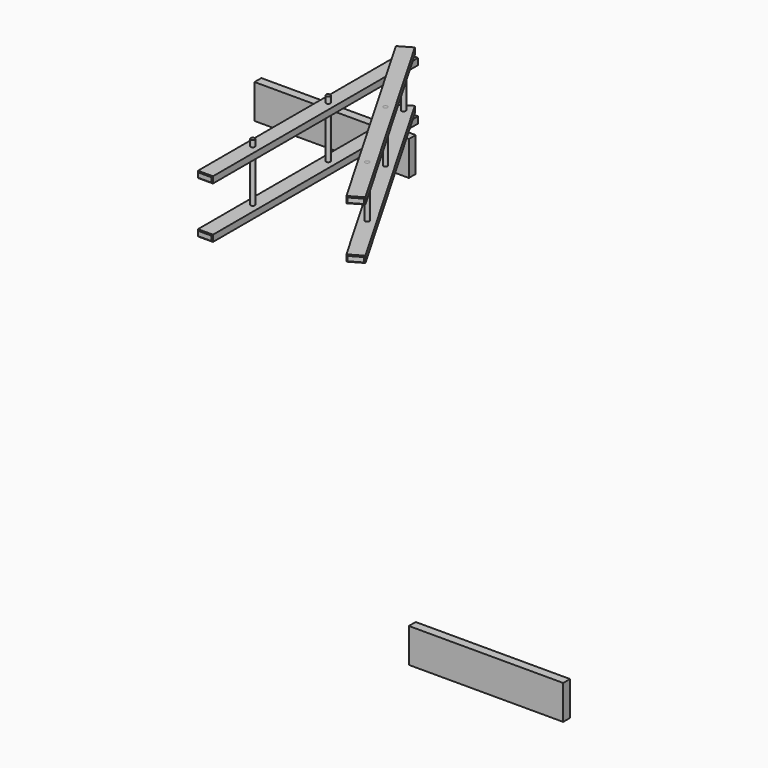
from build123d import *

# Parameters (mm, degrees)
F0_W      = 88.9
F0_H      = 38.1
F1_DEPTH  = 1524
F3_SIZE   = 5.08
F3_2_SIZE = 5.08
F4_R      = 12.7
F5_DEPTH  = 381
F6_ANGLE  = -30
F10_ANGLE = -30
F11_W     = 50.8
F11_H     = 203.2
F12_DEPTH = 914.4


with BuildPart() as f1:
    # F0 (on Front) → F1 (new body)
    with BuildSketch(Plane.XZ):
        with Locations((-209.1941202037, -63.0855914205)):
            Rectangle(F0_W, F0_H)
    extrude(amount=-F1_DEPTH)


with BuildPart() as f2_1:
    # F2: copy of F1
    add(f1.part.moved(Location((0, 0, 304.8))))

    # F3
    f3_edges = [f2_1.edges().sort_by_distance(p)[0] for p in [
        (-253.64412, 0, 241.714409),
        (-209.19412, 0, 222.664409),
        (-164.74412, 0, 241.714409),
        (-209.19412, 0, 260.764409),
    ]]
    chamfer(f3_edges, length=F3_SIZE)


with BuildPart() as f1_1:
    add(f1.part)

    # F3#2
    f3_2_edges = [f1_1.edges().sort_by_distance(p)[0] for p in [
        (-253.64412, 0, -63.085591),
        (-209.19412, 0, -82.135591),
        (-164.74412, 0, -63.085591),
        (-209.19412, 0, -44.035591),
    ]]
    chamfer(f3_2_edges, length=F3_2_SIZE)


with BuildPart() as f5:
    # F4 (on face) → F5 (new body)
    with BuildSketch(Plane(origin=(0, 0, -82.1355914205), x_dir=(1, 0, 0), z_dir=(0, 0, -1))):
        with Locations((-209.1941202037, -1473.2)):
            Circle(F4_R)
    extrude(amount=-F5_DEPTH)


with BuildPart() as f6_1:
    # F6: copy of F1
    add(f1_1.part.rotate(Axis((-209.1941202037, 1473.2, -82.1355914205), (0, 0, -1)), F6_ANGLE))


with BuildPart() as f6_2:
    # F6: copy of F2_1
    add(f2_1.part.rotate(Axis((-209.1941202037, 1473.2, -82.1355914205), (0, 0, -1)), F6_ANGLE))


with BuildPart() as f6_2_1:
    # F7: moved
    add(f6_2.part.moved(Location((0, 0, 38.1))))


with BuildPart() as f6_1_1:
    # F7: moved
    add(f6_1.part.moved(Location((0, 0, 38.1))))


with BuildPart() as f8_1:
    # F8: copy of F5
    add(f5.part.moved(Location((0, -558.8, 0))))


with BuildPart() as f9_1:
    # F9: copy of F8_1
    add(f8_1.part.moved(Location((0, -558.8, 0))))


with BuildPart() as f10_1:
    # F10: copy of F8_1
    add(f8_1.part.rotate(Axis((-209.1941202037, 1473.2, -82.1355914205), (0, 0, -1)), F10_ANGLE))


with BuildPart() as f10_2:
    # F10: copy of F9_1
    add(f9_1.part.rotate(Axis((-209.1941202037, 1473.2, -82.1355914205), (0, 0, -1)), F10_ANGLE))


with BuildPart() as f12:
    # F11 (on face) → F12 (new body)
    with BuildSketch(Plane(origin=(-253.6441202037, 0, 0), x_dir=(0, -1, 0), z_dir=(-1, 0, 0))):
        with Locations((-1592.443037352, -310.5422317326)):
            Rectangle(F11_W, F11_H)
    extrude(amount=F12_DEPTH)


with BuildPart() as f13_1:
    # F13: copy of F12
    add(f12.part.moved(Location((914.4, 0, 0))))


with BuildPart() as f13_1_1:
    # F14: moved
    add(f13_1.part.moved(Location((0, 0, -2540))))


solid = Compound([f2_1.part, f1_1.part, f5.part, f6_2_1.part, f6_1_1.part, f8_1.part, f9_1.part, f10_1.part, f10_2.part, f12.part, f13_1_1.part])
